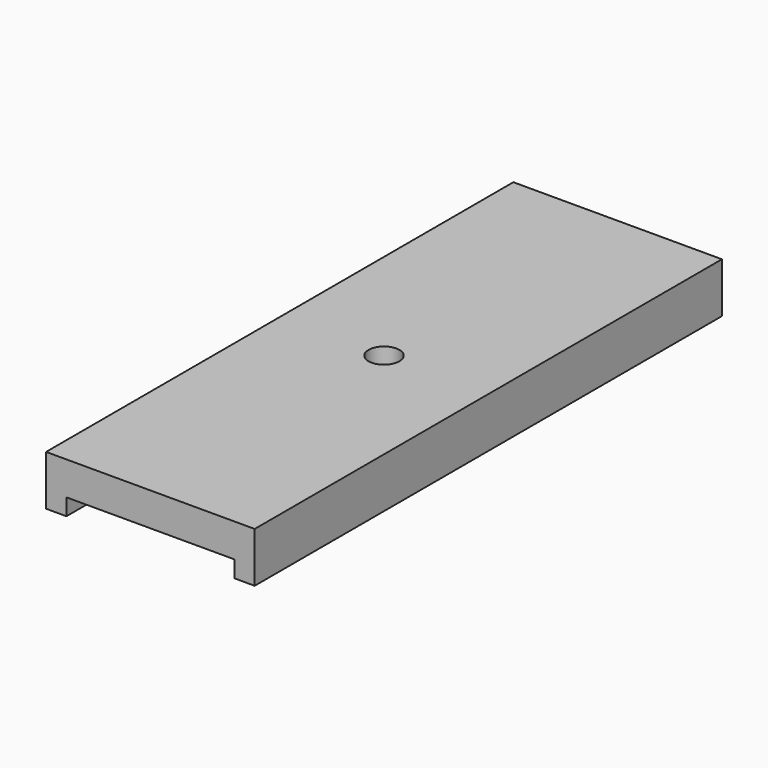
from build123d import *

# Parameters (mm, degrees)
F1_DEPTH = 35
F2_R     = 1.85
F3_DEPTH = 6.001


# Not quite as in the source:
# - a feature names something its author has since deleted; it is built from what else it names


with BuildPart() as f1:
    # F0 (on Front) → F1 (new body, symmetric)
    with BuildSketch(Plane.XZ):
        Polygon((-10.06, 8), (-10.06, 10), (10.06, 10), (10.06, 8), (12.5, 8), (12.5, 14), (-12.5, 14), (-12.5, 8), align=None)
    extrude(amount=F1_DEPTH, both=True)

    # F2 (on face) → F3 (cut, through all)
    with BuildSketch(Plane.XY.offset(14)):
        Circle(F2_R)
    extrude(amount=-F3_DEPTH, mode=Mode.SUBTRACT)


solid = f1.part
